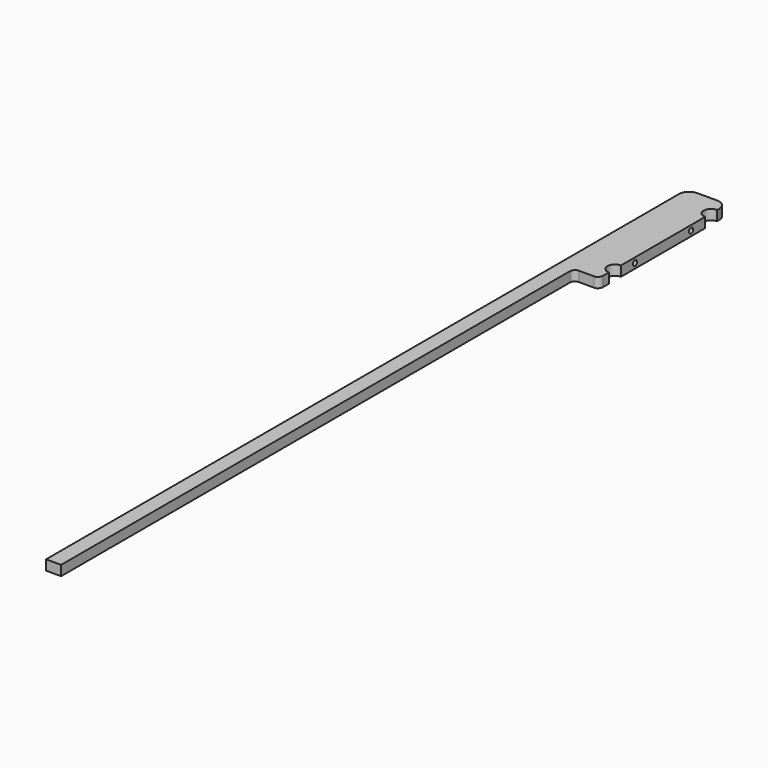
from build123d import *

# Parameters (mm, degrees)
F1_DEPTH = 12.7
F3_D     = 19.05
F5_D     = 6.5278
F5_DEPTH = 19.05
F5_TIP   = 1.9611489744


# Not quite as in the source:
# - a feature names something its author has since deleted; it is built from what else it names


with BuildPart() as f1:
    # F0 (on Top) → F1 (new body)
    with BuildSketch(Plane.XY):
        with BuildLine():
            Line((38.1, 1073.25354091), (12.7, 1073.25354091))
            ThreePointArc((12.7, 1073.25354091), (3.7197438789, 1069.5337970311), (0, 1060.55354091))
            Line((0, 1060.55354091), (0, 57.25354091))
            Line((0, 57.25354091), (19.05, 57.25354091))
            Line((19.05, 57.25354091), (19.05, 863.70354091))
            ThreePointArc((19.05, 863.70354091), (20.9098719395, 868.1936689706), (25.4, 870.05354091))
            Line((25.4, 870.05354091), (44.45, 870.05354091))
            ThreePointArc((44.45, 870.05354091), (48.9401280605, 871.9134128495), (50.8, 876.40354091))
            Line((50.8, 876.40354091), (50.8, 1060.55354091))
            ThreePointArc((50.8, 1060.55354091), (47.0802561211, 1069.5337970311), (38.1, 1073.25354091))
        make_face()
    extrude(amount=F1_DEPTH)

    # F3 (through all)
    with Locations(Plane.XY.offset(12.7)):
        with Locations((50.8, 1047.85354091), (50.8, 895.45354091)):
            Hole(F3_D / 2)

    # F5
    with Locations(Plane.YZ.offset(50.8)):
        with Locations((1016.10354091, 6.35), (927.20354091, 6.35)):
            Hole(F5_D / 2, depth=F5_DEPTH)
            with Locations((0, 0, -(F5_DEPTH + F5_TIP / 2))):  # 118° drill point
                Cone(0, F5_D / 2, F5_TIP, mode=Mode.SUBTRACT)


solid = f1.part
